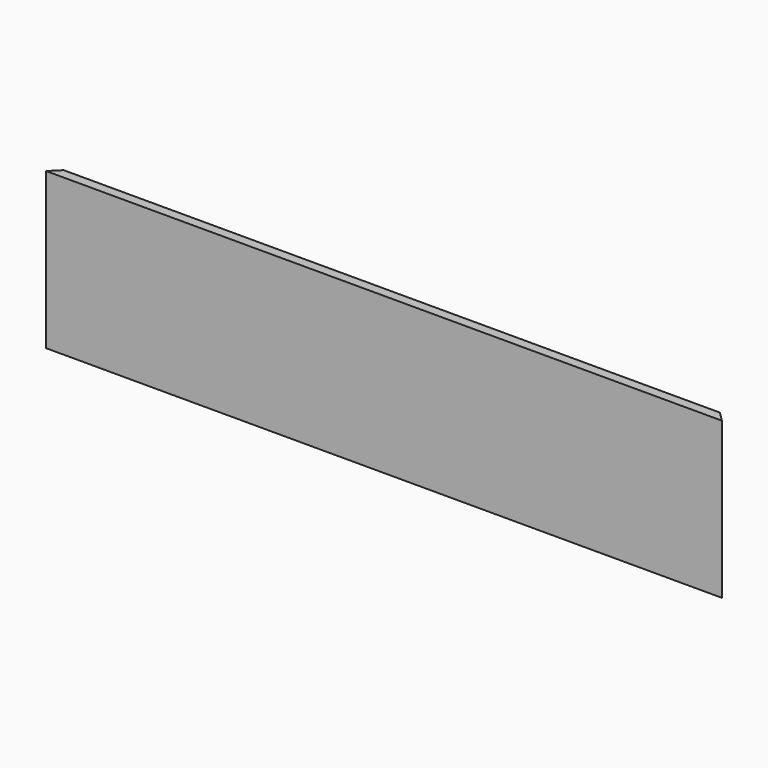
from build123d import *

# Parameters (mm, degrees)
F0_W     = 1320.8
F0_H     = 304.8
F1_DEPTH = 19.05
F2_SIZE  = 19.04999


# Not quite as in the source:
# - a fillet or chamfer is up to 0.001 mm smaller than in the source, because OpenCascade refuses the exact size


with BuildPart() as f1:
    # F0 (on Front) → F1 (new body)
    with BuildSketch(Plane.XZ):
        with Locations((332.2930652871, -11.7696728557)):
            Rectangle(F0_W, F0_H)
    extrude(amount=F1_DEPTH)

    # F2 (size 19.05 in the source; OpenCascade refuses exactly that, so slightly less here)
    f2_edges = [f1.edges().sort_by_distance(p)[0] for p in [
        (-328.106935, 0, -11.769673),
        (992.693065, 0, -11.769673),
    ]]
    chamfer(f2_edges, length=F2_SIZE)


solid = f1.part
